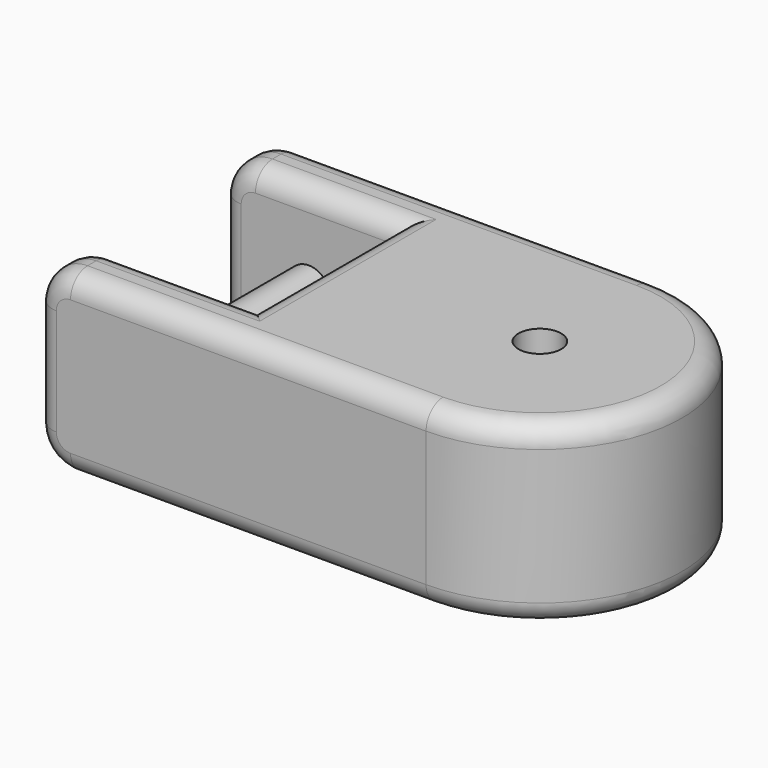
from build123d import *

# Parameters (mm, degrees)
F0_R         = 3
F1_DEPTH     = 12.5
F2_R         = 3
F3_DEPTH     = 40
F4_R         = 3
F5_T1_DEPTH  = 7.5
F5_T3_DEPTH  = 7.5
F5_T6_ANGLE  = 90
F5_T8_ANGLE  = 90
F5_T10_ANGLE = 90
F5_T12_ANGLE = 90
F5_T14_ANGLE = 90
F5_T16_ANGLE = 90
F5_T18_ANGLE = 90
F5_T20_ANGLE = 90


# Not quite as in the source:
# - a fillet or chamfer that OpenCascade refuses, or shapes differently, is made with other operations: its cross-section is extruded or revolved along the edge and cut away or added


with BuildPart() as f1:
    # F0 (on Top) → F1 (new body, symmetric)
    with BuildSketch(Plane.XY):
        with BuildLine():
            Line((-68.6048818245, -20), (-13.6048818245, -20))
            ThreePointArc((-13.6048818245, -20), (-33.6048818245, 0), (-13.6048818245, 20))
            Line((-13.6048818245, 20), (-68.6048818245, 20))
            Line((-68.6048818245, 20), (-68.6048818245, 12.5))
            Line((-68.6048818245, 12.5), (-43.6048818245, 12.5))
            Line((-43.6048818245, 12.5), (-43.6048818245, -12.5))
            Line((-43.6048818245, -12.5), (-68.6048818245, -12.5))
            Line((-68.6048818245, -12.5), (-68.6048818245, -20))
        make_face()
        with BuildLine():
            ThreePointArc((-13.6048818245, 20), (-33.6048818245, 0), (-13.6048818245, -20))
            ThreePointArc((-13.6048818245, -20), (0.5372537993, -14.1421356237), (6.3951181755, 0))
            ThreePointArc((6.3951181755, 0), (0.5372537993, 14.1421356237), (-13.6048818245, 20))
        make_face()
        with Locations((-13.6048818245, 0)):
            Circle(F0_R, mode=Mode.SUBTRACT)
    extrude(amount=F1_DEPTH, both=True)

    # F2 (on face) → F3 (join, through all)
    with BuildSketch(Plane.XZ.offset(20)):
        with Locations((-56.1048818245, 0)):
            Circle(F2_R)
    extrude(amount=-F3_DEPTH)

    # F4
    f4_edges = [f1.edges().sort_by_distance(p)[0] for p in [
        (-41.104882, 20, 12.5),
        (-43.604882, 0, 12.5),
        (-56.104882, 12.5, 12.5),
        (-56.104882, -12.5, 12.5),
        (6.395118, 0, -12.5),
        (-43.604882, 0, -12.5),
        (-68.604882, -12.5, 0),
        (-68.604882, 12.5, 0),
        (-56.104882, 12.5, -12.5),
        (-56.104882, -12.5, -12.5),
        (-68.604882, -20, 0),
        (-68.604882, 20, 0),
        (-41.104882, -20, -12.5),
        (-41.104882, -20, 12.5),
        (-41.104882, 20, -12.5),
        (6.395118, 0, 12.5),
    ]]
    fillet(f4_edges, radius=F4_R)

    # F5: fillet of radius 5 on 4 edges, made by hand

    # F5_s2 → F5_t1 (cut)
    with BuildSketch(Plane.XZ.offset(-20)):
        with BuildLine():
            ThreePointArc((-63.6048818245, 12.5), (-67.1404157304, 11.0355339059), (-68.6048818245, 7.5))
            Line((-68.6048818245, 7.5), (-68.6048818245, 12.5))
            Line((-68.6048818245, 12.5), (-63.6048818245, 12.5))
        make_face()
        with BuildLine():
            ThreePointArc((-63.6048818245, -12.5), (-67.1404157304, -11.0355339059), (-68.6048818245, -7.5))
            Line((-68.6048818245, -7.5), (-68.6048818245, -12.5))
            Line((-68.6048818245, -12.5), (-63.6048818245, -12.5))
        make_face()
    extrude(amount=F5_T1_DEPTH, mode=Mode.SUBTRACT)

    # F5_s4 → F5_t3 (cut)
    with BuildSketch(Plane.XZ.offset(12.5)):
        with BuildLine():
            ThreePointArc((-63.6048818245, -12.5), (-67.1404157304, -11.0355339059), (-68.6048818245, -7.5))
            Line((-68.6048818245, -7.5), (-68.6048818245, -12.5))
            Line((-68.6048818245, -12.5), (-63.6048818245, -12.5))
        make_face()
        with BuildLine():
            ThreePointArc((-63.6048818245, 12.5), (-67.1404157304, 11.0355339059), (-68.6048818245, 7.5))
            Line((-68.6048818245, 7.5), (-68.6048818245, 12.5))
            Line((-68.6048818245, 12.5), (-63.6048818245, 12.5))
        make_face()
    extrude(amount=F5_T3_DEPTH, mode=Mode.SUBTRACT)

    # F5_s5 → F5_t6 (revolve, cut)
    with BuildSketch(Plane.XY.offset(7.5)):
        with BuildLine():
            ThreePointArc((-65.6048818245, -12.5), (-67.726202168, -13.3786796564), (-68.6048818245, -15.5))
            Line((-68.6048818245, -15.5), (-68.6048818245, -12.5))
            Line((-68.6048818245, -12.5), (-65.6048818245, -12.5))
        make_face()
    revolve(axis=Axis((-63.6048818245, -12.5, 7.5), (0, 1, 0)), revolution_arc=F5_T6_ANGLE, mode=Mode.SUBTRACT)

    # F5_s7 → F5_t8 (revolve, cut)
    with BuildSketch(Plane.YZ.offset(-63.6048818245)):
        with BuildLine():
            ThreePointArc((-20, 9.5), (-19.1213203436, 11.6213203436), (-17, 12.5))
            Line((-17, 12.5), (-20, 12.5))
            Line((-20, 12.5), (-20, 9.5))
        make_face()
    revolve(axis=Axis((-63.6048818245, -20, 7.5), (0, -1, 0)), revolution_arc=F5_T8_ANGLE, mode=Mode.SUBTRACT)

    # F5_s9 → F5_t10 (revolve, cut)
    with BuildSketch(Plane.YZ.offset(-63.6048818245)):
        with BuildLine():
            ThreePointArc((-12.5, -9.5), (-13.3786796564, -11.6213203436), (-15.5, -12.5))
            Line((-15.5, -12.5), (-12.5, -12.5))
            Line((-12.5, -12.5), (-12.5, -9.5))
        make_face()
    revolve(axis=Axis((-63.6048818245, -12.5, -7.5), (0, 1, 0)), revolution_arc=F5_T10_ANGLE, mode=Mode.SUBTRACT)

    # F5_s11 → F5_t12 (revolve, cut)
    with BuildSketch(Plane.XY.offset(-7.5)):
        with BuildLine():
            ThreePointArc((-65.6048818245, -20), (-67.726202168, -19.1213203436), (-68.6048818245, -17))
            Line((-68.6048818245, -17), (-68.6048818245, -20))
            Line((-68.6048818245, -20), (-65.6048818245, -20))
        make_face()
    revolve(axis=Axis((-63.6048818245, -20, -7.5), (0, -1, 0)), revolution_arc=F5_T12_ANGLE, mode=Mode.SUBTRACT)

    # F5_s13 → F5_t14 (revolve, cut)
    with BuildSketch(Plane.YZ.offset(-63.6048818245)):
        with BuildLine():
            ThreePointArc((20, -9.5), (19.1213203436, -11.6213203436), (17, -12.5))
            Line((17, -12.5), (20, -12.5))
            Line((20, -12.5), (20, -9.5))
        make_face()
    revolve(axis=Axis((-63.6048818245, 20, -7.5), (0, 1, 0)), revolution_arc=F5_T14_ANGLE, mode=Mode.SUBTRACT)

    # F5_s15 → F5_t16 (revolve, cut)
    with BuildSketch(Plane.XY.offset(-7.5)):
        with BuildLine():
            ThreePointArc((-65.6048818245, 12.5), (-67.726202168, 13.3786796564), (-68.6048818245, 15.5))
            Line((-68.6048818245, 15.5), (-68.6048818245, 12.5))
            Line((-68.6048818245, 12.5), (-65.6048818245, 12.5))
        make_face()
    revolve(axis=Axis((-63.6048818245, 12.5, -7.5), (0, -1, 0)), revolution_arc=F5_T16_ANGLE, mode=Mode.SUBTRACT)

    # F5_s17 → F5_t18 (revolve, cut)
    with BuildSketch(Plane.XY.offset(7.5)):
        with BuildLine():
            ThreePointArc((-65.6048818245, 20), (-67.726202168, 19.1213203436), (-68.6048818245, 17))
            Line((-68.6048818245, 17), (-68.6048818245, 20))
            Line((-68.6048818245, 20), (-65.6048818245, 20))
        make_face()
    revolve(axis=Axis((-63.6048818245, 20, 7.5), (0, 1, 0)), revolution_arc=F5_T18_ANGLE, mode=Mode.SUBTRACT)

    # F5_s19 → F5_t20 (revolve, cut)
    with BuildSketch(Plane.YZ.offset(-63.6048818245)):
        with BuildLine():
            ThreePointArc((12.5, 9.5), (13.3786796564, 11.6213203436), (15.5, 12.5))
            Line((15.5, 12.5), (12.5, 12.5))
            Line((12.5, 12.5), (12.5, 9.5))
        make_face()
    revolve(axis=Axis((-63.6048818245, 12.5, 7.5), (0, -1, 0)), revolution_arc=F5_T20_ANGLE, mode=Mode.SUBTRACT)


solid = f1.part
